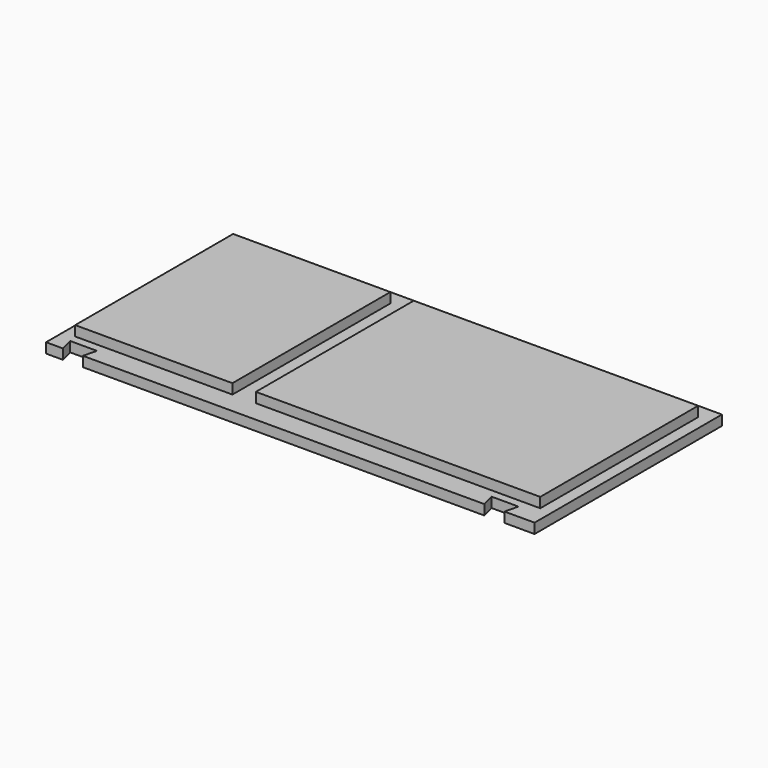
from build123d import *

# Parameters (mm, degrees)
F0_W         = 146
F0_H         = 70
F1_DEPTH     = 3
F2_W         = 47
F2_H         = 59
F2_W_2       = 85
F3_DEPTH     = 3
F4_DEPTH     = 3
F5_DEPTH     = 3
F6_TEXT_SIZE = 14.0588388441
F7_DEPTH     = 2


# Not quite as in the source:
# - Text() gives the source's letters only with a copy of the font that has no kerning and outlines rounded to 1/6400 em; it was checked with that copy


with BuildPart() as f1:
    # F0 (on Top) → F1 (new body)
    with BuildSketch(Plane.XY):
        with Locations((73, 35)):
            Rectangle(F0_W, F0_H)
    extrude(amount=F1_DEPTH)

    # F2 (on face) → F3 (join)
    with BuildSketch(Plane.XY.offset(3)):
        with Locations((27, 36)):
            Rectangle(F2_W, F2_H)
        with Locations((100, 36)):
            Rectangle(F2_W_2, F2_H)
    extrude(amount=F3_DEPTH)

    # F2 (on face) → F4 (cut)
    with BuildSketch(Plane.XY.offset(3)):
        Polygon((12, 4), (4, 4), (5, 0), (11, 0), align=None)
    extrude(amount=-F4_DEPTH, mode=Mode.SUBTRACT)

    # F2 (on face) → F5 (cut)
    with BuildSketch(Plane.XY.offset(3)):
        Polygon((138, 4), (130, 4), (131, 0), (137, 0), align=None)
    extrude(amount=-F5_DEPTH, mode=Mode.SUBTRACT)

    # F6 (on face) → F7 (join)
    with BuildSketch(Plane(origin=(0, 0, 0), x_dir=(1, 0, 0), z_dir=(0, 0, -1))):
        with Locations(Location((139.9923367626, -43.029036036), (0, 0, -180))):
            Text('iGEM Grenoble 2017', F6_TEXT_SIZE, font='Open Sans', text_align=(TextAlign.LEFT, TextAlign.BOTTOM))
        with Locations(Location((103.4613227038, -23.9090152081), (0, 0, -180))):
            Text('SnapLab', F6_TEXT_SIZE, font='Open Sans', text_align=(TextAlign.LEFT, TextAlign.BOTTOM))
    extrude(amount=F7_DEPTH)


solid = f1.part
